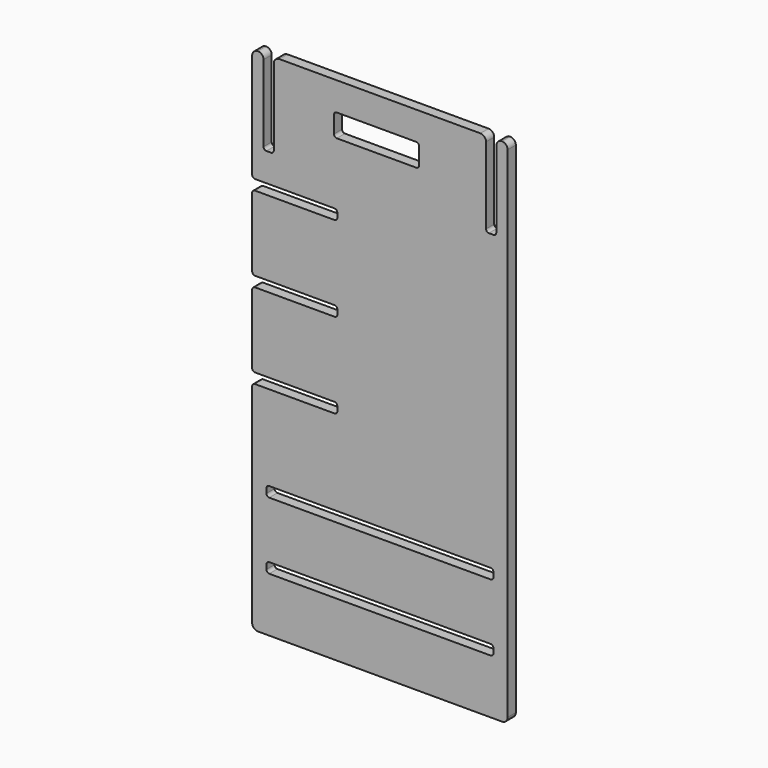
from build123d import *

# Parameters (mm, degrees)
F1_DEPTH  = 18
F2_W      = 400
F2_H      = 18
F3_DEPTH  = 25
F4_W      = 400
F4_H      = 18
F5_DEPTH  = 25
F6_R      = 10
F7_R      = 10
F8_R      = 9.99999
F9_R      = 5
F10_R     = 5
F11_R     = 5
F12_W     = 150
F12_H     = 40
F13_DEPTH = 25
F14_R     = 5


# Not quite as in the source:
# - a fillet or chamfer is up to 0.001 mm smaller than in the source, because OpenCascade refuses the exact size


with BuildPart() as f1:
    # F0 (on Front) → F1 (new body)
    with BuildSketch(Plane.XZ):
        Polygon((0, 382), (0, 0), (450, 0), (450, 900), (430, 900), (430, 750), (412, 750), (412, 900), (38, 900), (38, 750), (20, 750), (20, 900), (0, 900), (0, 700), (150, 700), (150, 682), (0, 682), (0, 550), (150, 550), (150, 532), (0, 532), (0, 400), (150, 400), (150, 382), align=None)
    extrude(amount=F1_DEPTH)

    # F2 (on face) → F3 (cut)
    with BuildSketch(Plane.XZ.offset(18)):
        with Locations((225, 223)):
            Rectangle(F2_W, F2_H)
    extrude(amount=-F3_DEPTH, mode=Mode.SUBTRACT)

    # F4 (on face) → F5 (cut)
    with BuildSketch(Plane.XZ.offset(18)):
        with Locations((225, 105)):
            Rectangle(F4_W, F4_H)
    extrude(amount=-F5_DEPTH, mode=Mode.SUBTRACT)

    # F6
    f6_edges = [f1.edges().sort_by_distance(p)[0] for p in [
        (450, -9, 0),
    ]]
    fillet(f6_edges, radius=F6_R)

    # F7
    f7_edges = [f1.edges().sort_by_distance(p)[0] for p in [
        (0, -9, 0),
    ]]
    fillet(f7_edges, radius=F7_R)

    # F8 (radius 10 in the source; OpenCascade refuses exactly that, so slightly less here)
    f8_edges = [f1.edges().sort_by_distance(p)[0] for p in [
        (450, -9, 900),
        (430, -9, 900),
        (412, -9, 900),
        (38, -9, 900),
        (20, -9, 900),
        (0, -9, 900),
    ]]
    fillet(f8_edges, radius=F8_R)

    # F9
    f9_edges = [f1.edges().sort_by_distance(p)[0] for p in [
        (0, -9, 382),
        (0, -9, 400),
        (0, -9, 532),
        (0, -9, 550),
        (0, -9, 682),
        (0, -9, 700),
    ]]
    fillet(f9_edges, radius=F9_R)

    # F10
    f10_edges = [f1.edges().sort_by_distance(p)[0] for p in [
        (25, -9, 232),
        (25, -9, 214),
        (25, -9, 96),
        (25, -9, 114),
        (425, -9, 114),
        (425, -9, 96),
        (425, -9, 214),
        (425, -9, 232),
    ]]
    fillet(f10_edges, radius=F10_R)

    # F11
    f11_edges = [f1.edges().sort_by_distance(p)[0] for p in [
        (150, -9, 382),
        (150, -9, 400),
        (150, -9, 532),
        (150, -9, 550),
        (150, -9, 700),
        (150, -9, 682),
        (38, -9, 750),
        (20, -9, 750),
        (412, -9, 750),
        (430, -9, 750),
    ]]
    fillet(f11_edges, radius=F11_R)

    # F12 (on face) → F13 (cut)
    with BuildSketch(Plane.XZ.offset(18)):
        with Locations((219, 830)):
            Rectangle(F12_W, F12_H)
    extrude(amount=-F13_DEPTH, mode=Mode.SUBTRACT)

    # F14
    f14_edges = [f1.edges().sort_by_distance(p)[0] for p in [
        (144, -9, 810),
        (144, -9, 850),
        (294, -9, 850),
        (294, -9, 810),
    ]]
    fillet(f14_edges, radius=F14_R)


solid = f1.part
